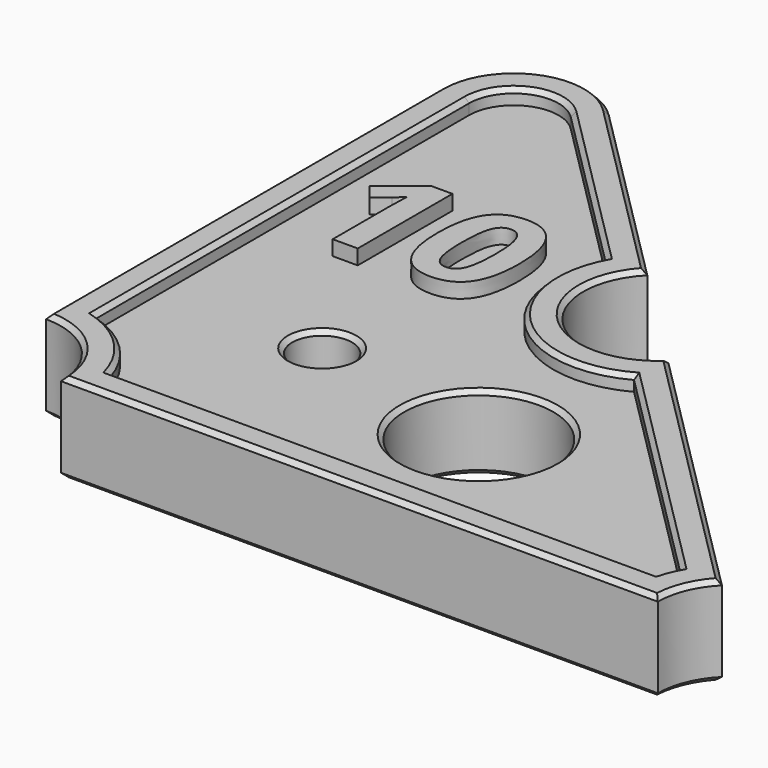
from build123d import *

# Parameters (mm, degrees)
F0_R         = 2
F0_R_2       = 5
F0_TEXT_SIZE = 11.1111111111
F1_DEPTH     = 5
F3_DEPTH     = 1
F4_SIZE      = 0.3


# Not quite as in the source:
# - Text() gives the source's letters only with a copy of the font that has no kerning and outlines rounded to 1/6400 em; it was checked with that copy


with BuildPart() as f1:
    # F0 (on Top) → F1 (new body)
    with BuildSketch(Plane.XY):
        with BuildLine():
            ThreePointArc((-16.4644660941, 16.4644660941), (-21.9134171618, 17.5483298507), (-25, 12.9289321881))
            Line((-25, 12.9289321881), (-25, -20))
            ThreePointArc((-25, -20), (-21.4644660941, -21.4644660941), (-20, -25))
            Line((-20, -25), (20, -25))
            ThreePointArc((20, -25), (20.3806023374, -23.0865828382), (21.4644660941, -21.4644660941))
            Line((21.4644660941, -21.4644660941), (3.5355339059, -3.5355339059))
            ThreePointArc((3.5355339059, -3.5355339059), (-3.5355339059, -3.5355339059), (-3.5355339059, 3.5355339059))
            Line((-3.5355339059, 3.5355339059), (-16.4644660941, 16.4644660941))
        make_face()
        with Locations((-12.5, -12.5)):
            Circle(F0_R, mode=Mode.SUBTRACT)
        with Locations((0, -15)):
            Circle(F0_R_2, mode=Mode.SUBTRACT)
        with BuildLine():
            Line((-16.9140625, 3.9322916667), (-16.9140625, -4))
            Line((-16.9140625, -4), (-18.5911458333, -4))
            Line((-18.5911458333, -4), (-18.5911458333, 0.5902777778))
            Line((-18.5911458333, 0.5902777778), (-18.5737847222, 1.34375))
            Line((-18.5737847222, 1.34375), (-18.5477430556, 2.1684027778))
            add(Edge.make_bspline(
                [(-18.5477430556, 2.1684027778), (-18.9644097222, 1.7517361111), (-19.1276041667, 1.6215277778)],
                knots=[0, 0, 0, 1, 1, 1], degree=2))
            Line((-19.1276041667, 1.6215277778), (-20.0390625, 0.8888888889))
            Line((-20.0390625, 0.8888888889), (-20.8480902778, 1.8975694444))
            Line((-20.8480902778, 1.8975694444), (-18.2925347222, 3.9322916667))
            Line((-18.2925347222, 3.9322916667), (-16.9140625, 3.9322916667))
        make_face(mode=Mode.SUBTRACT)
        with BuildLine():
            add(Edge.make_bspline(
                [(-9.9184027778, 3.015625), (-9.2161458333, 1.9739583333), (-9.2161458333, -0.0347222222)],
                knots=[0, 0, 0, 1, 1, 1], degree=2))
            add(Edge.make_bspline(
                [(-9.2161458333, -0.0347222222), (-9.2161458333, -2.1111111111), (-9.8967013889, -3.1102430556)],
                knots=[0, 0, 0, 1, 1, 1], degree=2))
            add(Edge.make_bspline(
                [(-9.8967013889, -3.1102430556), (-10.5772569444, -4.109375), (-11.9939236111, -4.109375)],
                knots=[0, 0, 0, 1, 1, 1], degree=2))
            add(Edge.make_bspline(
                [(-11.9939236111, -4.109375), (-13.3671875, -4.109375), (-14.0642361111, -3.078125)],
                knots=[0, 0, 0, 1, 1, 1], degree=2))
            add(Edge.make_bspline(
                [(-14.0642361111, -3.078125), (-14.7612847222, -2.046875), (-14.7612847222, -0.0347222222)],
                knots=[0, 0, 0, 1, 1, 1], degree=2))
            add(Edge.make_bspline(
                [(-14.7612847222, -0.0347222222), (-14.7612847222, 2.0659722222), (-14.0824652778, 3.0616319444)],
                knots=[0, 0, 0, 1, 1, 1], degree=2))
            add(Edge.make_bspline(
                [(-14.0824652778, 3.0616319444), (-13.4036458333, 4.0572916667), (-11.9939236111, 4.0572916667)],
                knots=[0, 0, 0, 1, 1, 1], degree=2))
            add(Edge.make_bspline(
                [(-11.9939236111, 4.0572916667), (-10.6206597222, 4.0572916667), (-9.9184027778, 3.015625)],
                knots=[0, 0, 0, 1, 1, 1], degree=2))
        make_face(mode=Mode.SUBTRACT)
        with Locations((-21.5043402778, -4)):
            Text('10', F0_TEXT_SIZE, font='Open Sans', font_style=FontStyle.BOLD, text_align=(TextAlign.LEFT, TextAlign.BOTTOM))
        with BuildLine():
            add(Edge.make_bspline(
                [(-12.8402777778, 2.0625), (-13.0946180556, 1.4253472222), (-13.0946180556, -0.0347222222)],
                knots=[0, 0, 0, 1, 1, 1], degree=2))
            add(Edge.make_bspline(
                [(-13.0946180556, -0.0347222222), (-13.0946180556, -1.4930555556), (-12.8428819444, -2.125)],
                knots=[0, 0, 0, 1, 1, 1], degree=2))
            add(Edge.make_bspline(
                [(-12.8428819444, -2.125), (-12.5911458333, -2.7569444444), (-11.9939236111, -2.7569444444)],
                knots=[0, 0, 0, 1, 1, 1], degree=2))
            add(Edge.make_bspline(
                [(-11.9939236111, -2.7569444444), (-11.4071180556, -2.7569444444), (-11.1467013889, -2.1171875)],
                knots=[0, 0, 0, 1, 1, 1], degree=2))
            add(Edge.make_bspline(
                [(-11.1467013889, -2.1171875), (-10.8862847222, -1.4774305556), (-10.8862847222, -0.0347222222)],
                knots=[0, 0, 0, 1, 1, 1], degree=2))
            add(Edge.make_bspline(
                [(-10.8862847222, -0.0347222222), (-10.8862847222, 1.4253472222), (-11.1501736111, 2.0625)],
                knots=[0, 0, 0, 1, 1, 1], degree=2))
            add(Edge.make_bspline(
                [(-11.1501736111, 2.0625), (-11.4140625, 2.6996527778), (-11.9939236111, 2.6996527778)],
                knots=[0, 0, 0, 1, 1, 1], degree=2))
            add(Edge.make_bspline(
                [(-11.9939236111, 2.6996527778), (-12.5859375, 2.6996527778), (-12.8402777778, 2.0625)],
                knots=[0, 0, 0, 1, 1, 1], degree=2))
        make_face()
    extrude(amount=-F1_DEPTH)

    # F0 (on Top) + F2 (on face) → F3 (join)
    with BuildSketch(Plane.XY):
        with Locations((-21.5043402778, -4)):
            Text('10', F0_TEXT_SIZE, font='Open Sans', font_style=FontStyle.BOLD, text_align=(TextAlign.LEFT, TextAlign.BOTTOM))
    with BuildSketch(Plane.XY):
        with BuildLine():
            ThreePointArc((20, -25), (20.3806023374, -23.0865828382), (21.4644660941, -21.4644660941))
            Line((21.4644660941, -21.4644660941), (3.5355339059, -3.5355339059))
            ThreePointArc((3.5355339059, -3.5355339059), (-3.5355339059, -3.5355339059), (-3.5355339059, 3.5355339059))
            Line((-3.5355339059, 3.5355339059), (-16.4644660941, 16.4644660941))
            ThreePointArc((-16.4644660941, 16.4644660941), (-21.9134171618, 17.5483298507), (-25, 12.9289321881))
            Line((-25, 12.9289321881), (-25, -20))
            ThreePointArc((-25, -20), (-21.4644660941, -21.4644660941), (-20, -25))
            Line((-20, -25), (20, -25))
        make_face()
        with BuildLine():
            Line((3.3292029279, -6.1576300526), (18.8423699474, -21.6707970721))
            ThreePointArc((18.8423699474, -21.6707970721), (18.5328432724, -22.3212159734), (18.2917960675, -23))
            Line((18.2917960675, -23), (-18.2917960675, -23))
            ThreePointArc((-18.2917960675, -23), (-20.0502525317, -20.0502525317), (-23, -18.2917960675))
            Line((-23, -18.2917960675), (-23, 12.9289321881))
            ThreePointArc((-23, 12.9289321881), (-21.1480502971, 15.7005707857), (-17.8786796564, 15.0502525317))
            Line((-17.8786796564, 15.0502525317), (-6.1576300526, 3.3292029279))
            ThreePointArc((-6.1576300526, 3.3292029279), (-4.9497474683, -4.9497474683), (3.3292029279, -6.1576300526))
        make_face(mode=Mode.SUBTRACT)
    extrude(amount=F3_DEPTH)

    # F4
    f4_edges = [f1.edges().sort_by_distance(p)[0] for p in [
        (-14.5, -12.5, 0),
        (-5, -15, 0),
        (-21.464466, -21.464466, 1),
        (0, -25, 1),
        (20.380602, -23.086583, 1),
        (12.5, -12.5, 1),
        (-3.535534, -3.535534, 1),
        (-10, 10, 1),
        (-21.913417, 17.54833, 1),
        (-25, -3.535534, 1),
        (-12.018155, 9.189728, 1),
        (-4.949747, -4.949747, 1),
        (11.085786, -13.914214, 1),
        (18.532843, -22.321216, 1),
        (0, -23, 1),
        (-20.050253, -20.050253, 1),
        (-23, -2.681432, 1),
        (-21.14805, 15.700571, 1),
        (12.5, -12.5, -5),
        (-3.535534, -3.535534, -5),
        (-10, 10, -5),
        (-21.913417, 17.54833, -5),
        (-25, -3.535534, -5),
        (-21.464466, -21.464466, -5),
        (0, -25, -5),
        (20.380602, -23.086583, -5),
        (-14.5, -12.5, -5),
        (-5, -15, -5),
    ]]
    chamfer(f4_edges, length=F4_SIZE)


solid = f1.part
